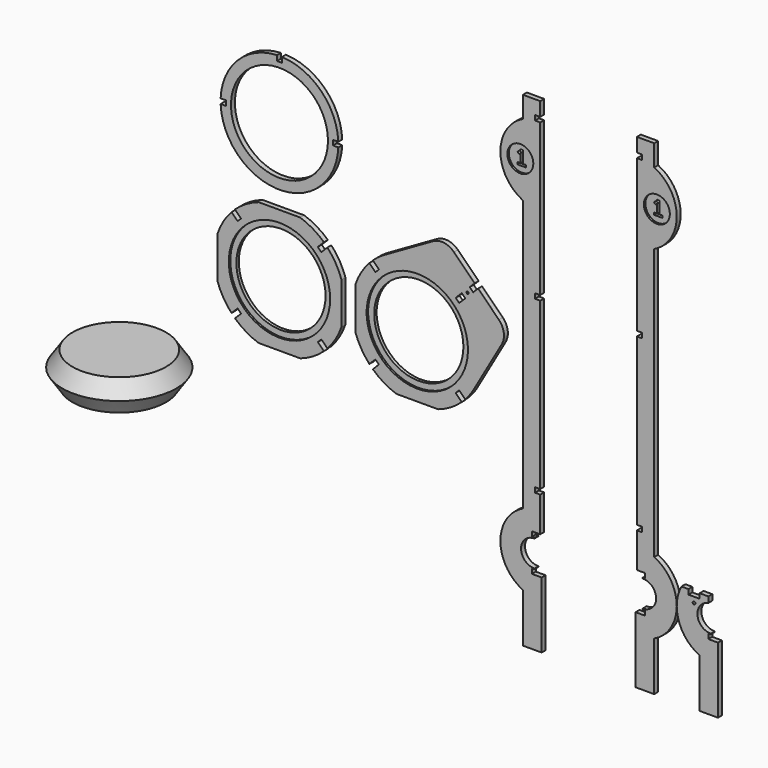
from build123d import *

# Parameters (mm, degrees)
F1_R     = 177.8
F2_DEPTH = 18.034
F1_R_2   = 185.7375
F1_R_3   = 3.81
F1_R_4   = 47.625
F1_W     = 5.08
F1_H     = 242.316
F1_R_5   = 5.08
F1_R_6   = 163.5125
F3_DEPTH = 11.176
F1_W_2   = 171.45
F1_H_2   = 114.3


# Not quite as in the source:
# - a variable given as a bare number and used for a length is read in inches; the dataset says mm whatever the document's units were
# - a feature names something its author has since deleted; it is built from what else it names


with BuildPart() as f2:
    # F1 (on Front) → F2 (new body)
    with BuildSketch(Plane.XZ):
        with BuildLine():
            Line((196.661621641, 517.017), (215.711621641, 517.017))
            ThreePointArc((215.711621641, 517.017), (152.6643540582, 660.6643540582), (9.017, 723.711621641))
            Line((9.017, 723.711621641), (9.017, 704.661621641))
            Line((9.017, 704.661621641), (-9.017, 704.661621641))
            Line((-9.017, 704.661621641), (-9.017, 723.711621641))
            ThreePointArc((-9.017, 723.711621641), (-152.6643540582, 660.6643540582), (-215.711621641, 517.017))
            Line((-215.711621641, 517.017), (-196.661621641, 517.017))
            Line((-196.661621641, 517.017), (-196.661621641, 498.983))
            Line((-196.661621641, 498.983), (-215.711621641, 498.983))
            ThreePointArc((-215.711621641, 498.983), (0, 292.1), (215.711621641, 498.983))
            Line((215.711621641, 498.983), (196.661621641, 498.983))
            Line((196.661621641, 498.983), (196.661621641, 517.017))
        make_face()
        with Locations((0, 508)):
            Circle(F1_R, mode=Mode.SUBTRACT)
    extrude(amount=F2_DEPTH)


with BuildPart() as f2b:
    # F1 (on Front) → F2, piece 2 (new body)
    with BuildSketch(Plane.XZ):
        with BuildLine():
            Line((76.2, 227.2787773996), (-76.2, 227.2787773996))
            ThreePointArc((-76.2, 227.2787773996), (-122.3458738565, 206.1396851811), (-163.0063908604, 175.7583545523))
            Line((-163.0063908604, 175.7583545523), (-140.6757121365, 153.4276758285))
            Line((-140.6757121365, 153.4276758285), (-153.4276758285, 140.6757121365))
            Line((-153.4276758285, 140.6757121365), (-175.7583545523, 163.0063908604))
            ThreePointArc((-175.7583545523, 163.0063908604), (-206.1396851811, 122.3458738565), (-227.2787773996, 76.2))
            Line((-227.2787773996, 76.2), (-227.2787773996, -76.2))
            ThreePointArc((-227.2787773996, -76.2), (-206.1396851811, -122.3458738565), (-175.7583545523, -163.0063908604))
            Line((-175.7583545523, -163.0063908604), (-153.4276758285, -140.6757121365))
            Line((-153.4276758285, -140.6757121365), (-140.6757121365, -153.4276758285))
            Line((-140.6757121365, -153.4276758285), (-163.0063908604, -175.7583545523))
            ThreePointArc((-163.0063908604, -175.7583545523), (-122.3458738565, -206.1396851811), (-76.2, -227.2787773996))
            Line((-76.2, -227.2787773996), (76.2, -227.2787773996))
            ThreePointArc((76.2, -227.2787773996), (122.3458738565, -206.1396851811), (163.0063908604, -175.7583545523))
            Line((163.0063908604, -175.7583545523), (140.6757121365, -153.4276758285))
            Line((140.6757121365, -153.4276758285), (153.4276758285, -140.6757121365))
            Line((153.4276758285, -140.6757121365), (175.7583545523, -163.0063908604))
            ThreePointArc((175.7583545523, -163.0063908604), (206.1396851811, -122.3458738565), (227.2787773996, -76.2))
            Line((227.2787773996, -76.2), (227.2787773996, 76.2))
            ThreePointArc((227.2787773996, 76.2), (206.1396851811, 122.3458738565), (175.7583545523, 163.0063908604))
            Line((175.7583545523, 163.0063908604), (153.4276758285, 140.6757121365))
            Line((153.4276758285, 140.6757121365), (140.6757121365, 153.4276758285))
            Line((140.6757121365, 153.4276758285), (163.0063908604, 175.7583545523))
            ThreePointArc((163.0063908604, 175.7583545523), (122.3458738565, 206.1396851811), (76.2, 227.2787773996))
        make_face()
        Circle(F1_R_2, mode=Mode.SUBTRACT)
    extrude(amount=F2_DEPTH)

    # F1 (on Front) → F3 (join)
    with BuildSketch(Plane.XZ):
        Circle(F1_R_2)
        Circle(F1_R_6, mode=Mode.SUBTRACT)
    extrude(amount=F3_DEPTH)


with BuildPart() as f2c:
    # F1 (on Front) → F2, piece 3 (new body)
    with BuildSketch(Plane.XZ):
        with BuildLine():
            Line((646.0332669357, -153.4276758285), (658.7852306276, -140.6757121365))
            Line((658.7852306276, -140.6757121365), (681.1159093515, -163.0063908604))
            ThreePointArc((681.1159093515, -163.0063908604), (701.321703842, -138.0584475726), (718.0125690949, -110.6342060628))
            ThreePointArc((718.0125690949, -110.6342060628), (725.9972246359, -93.7028214656), (732.6363321988, -76.2))
            Line((732.6363321988, -76.2), (732.6363321988, 76.2))
            ThreePointArc((732.6363321988, 76.2), (711.4972399802, 122.3458738565), (681.1159093515, 163.0063908604))
            Line((681.1159093515, 163.0063908604), (658.7852306276, 140.6757121365))
            Line((658.7852306276, 140.6757121365), (646.0332669357, 153.4276758285))
            Line((646.0332669357, 153.4276758285), (668.3639456595, 175.7583545523))
            ThreePointArc((668.3639456595, 175.7583545523), (627.7034286556, 206.1396851811), (581.5575547992, 227.2787773996))
            Line((581.5575547992, 227.2787773996), (429.1575547992, 227.2787773996))
            ThreePointArc((429.1575547992, 227.2787773996), (411.6547333336, 220.6396698367), (394.7233487364, 212.6550142957))
            ThreePointArc((394.7233487364, 212.6550142957), (367.2991072265, 195.9641490428), (342.3511639388, 175.7583545523))
            Line((342.3511639388, 175.7583545523), (364.6818426626, 153.4276758285))
            Line((364.6818426626, 153.4276758285), (351.9298789707, 140.6757121365))
            Line((351.9298789707, 140.6757121365), (329.5992002469, 163.0063908604))
            ThreePointArc((329.5992002469, 163.0063908604), (299.2178696181, 122.3458738565), (278.0787773996, 76.2))
            Line((278.0787773996, 76.2), (278.0787773996, -76.2))
            ThreePointArc((278.0787773996, -76.2), (299.2178696181, -122.3458738565), (329.5992002469, -163.0063908604))
            Line((329.5992002469, -163.0063908604), (351.9298789707, -140.6757121365))
            Line((351.9298789707, -140.6757121365), (364.6818426626, -153.4276758285))
            Line((364.6818426626, -153.4276758285), (342.3511639388, -175.7583545523))
            ThreePointArc((342.3511639388, -175.7583545523), (383.0116809427, -206.1396851811), (429.1575547992, -227.2787773996))
            Line((429.1575547992, -227.2787773996), (581.5575547992, -227.2787773996))
            ThreePointArc((581.5575547992, -227.2787773996), (627.7034286556, -206.1396851811), (668.3639456595, -175.7583545523))
            Line((668.3639456595, -175.7583545523), (646.0332669357, -153.4276758285))
        make_face()
        with Locations((505.3575547992, 0)):
            Circle(F1_R_2, mode=Mode.SUBTRACT)
        with BuildLine():
            ThreePointArc((732.6363321988, -76.2), (725.9972246359, -93.7028214656), (718.0125690949, -110.6342060628))
            Line((718.0125690949, -110.6342060628), (814.5833852283, 57.7646913023))
            ThreePointArc((814.5833852283, 57.7646913023), (822.4429089781, 97.7343199195), (804.399605341, 134.2553072998))
            Line((804.399605341, 134.2553072998), (728.3822155659, 210.2726970748))
            Line((728.3822155659, 210.2726970748), (710.3017417449, 192.1922232538))
            Line((710.3017417449, 192.1922232538), (697.549778053, 204.9441869458))
            Line((697.549778053, 204.9441869458), (715.630251874, 223.0246607668))
            Line((715.630251874, 223.0246607668), (639.612862099, 299.0420505418))
            ThreePointArc((639.612862099, 299.0420505418), (603.0918747187, 317.085354179), (563.1222461014, 309.2258304291))
            Line((563.1222461014, 309.2258304291), (394.7233487364, 212.6550142957))
            ThreePointArc((394.7233487364, 212.6550142957), (411.6547333336, 220.6396698367), (429.1575547992, 227.2787773996))
            Line((429.1575547992, 227.2787773996), (581.5575547992, 227.2787773996))
            ThreePointArc((581.5575547992, 227.2787773996), (627.7034286556, 206.1396851811), (668.3639456595, 175.7583545523))
            ThreePointArc((668.3639456595, 175.7583545523), (674.8598890843, 169.5023342852), (681.1159093515, 163.0063908604))
            ThreePointArc((681.1159093515, 163.0063908604), (711.4972399802, 122.3458738565), (732.6363321988, 76.2))
            Line((732.6363321988, 76.2), (732.6363321988, -76.2))
        make_face()
        with Locations((689.3928244917, 184.0352696925)):
            Circle(F1_R_3, mode=Mode.SUBTRACT)
    extrude(amount=F2_DEPTH)

    # F1 (on Front) → F3, piece 2 (join)
    with BuildSketch(Plane.XZ):
        with Locations((505.3575547992, 0)):
            Circle(F1_R_2)
        with Locations((505.3575547992, 0)):
            Circle(F1_R_6, mode=Mode.SUBTRACT)
    extrude(amount=F3_DEPTH)


with BuildPart() as f2d:
    # F1 (on Front) → F2, piece 4 (new body)
    with BuildSketch(Plane.XZ):
        with BuildLine():
            Line((1373.9863321988, 889), (1310.4863321988, 889))
            Line((1310.4863321988, 889), (1310.4863321988, 838.2))
            Line((1310.4863321988, 838.2), (1329.5363321988, 838.2))
            Line((1329.5363321988, 838.2), (1329.5363321988, 820.166))
            Line((1329.5363321988, 820.166), (1310.4863321988, 820.166))
            Line((1310.4863321988, 820.166), (1310.4863321988, 263.017))
            Line((1310.4863321988, 263.017), (1329.5363321988, 263.017))
            Line((1329.5363321988, 263.017), (1329.5363321988, 244.983))
            Line((1329.5363321988, 244.983), (1310.4863321988, 244.983))
            Line((1310.4863321988, 244.983), (1310.4863321988, -362.966))
            Line((1310.4863321988, -362.966), (1329.5363321988, -362.966))
            Line((1329.5363321988, -362.966), (1329.5363321988, -381))
            Line((1329.5363321988, -381), (1310.4863321988, -381))
            Line((1310.4863321988, -381), (1310.4863321988, -487.934))
            Line((1310.4863321988, -487.934), (1310.4863321988, -509.016))
            Line((1310.4863321988, -509.016), (1340.8367921988, -509.016))
            Line((1340.8367921988, -509.016), (1340.8367921988, -527.05))
            Line((1340.8367921988, -527.05), (1331.7029521988, -527.05))
            Line((1331.7029521988, -527.05), (1331.7029521988, -529.6289769048))
            ThreePointArc((1331.7029521988, -529.6289769048), (1380.8443321988, -577.85), (1331.7029521988, -626.0710230952))
            Line((1331.7029521988, -626.0710230952), (1331.7029521988, -628.65))
            Line((1331.7029521988, -628.65), (1340.8367921988, -628.65))
            Line((1340.8367921988, -628.65), (1340.8367921988, -646.684))
            Line((1340.8367921988, -646.684), (1310.4863321988, -646.684))
            Line((1310.4863321988, -646.684), (1310.4863321988, -889))
            Line((1310.4863321988, -889), (1373.9863321988, -889))
            Line((1373.9863321988, -889), (1373.9863321988, -709.3732013753))
            ThreePointArc((1373.9863321988, -709.3732013753), (1434.18915654, -655.491572305), (1456.5363321988, -577.85))
            ThreePointArc((1456.5363321988, -577.85), (1434.18915654, -500.208427695), (1373.9863321988, -446.3267986247))
            Line((1373.9863321988, -446.3267986247), (1373.9863321988, 547.9267986247))
            ThreePointArc((1373.9863321988, 547.9267986247), (1456.5363321988, 679.45), (1373.9863321988, 810.9732013753))
            Line((1373.9863321988, 810.9732013753), (1373.9863321988, 889))
        make_face()
        with Locations((1383.5113321988, 679.45)):
            Circle(F1_R_4, mode=Mode.SUBTRACT)
        with Locations((1307.9463321988, -767.842)):
            Rectangle(F1_W, F1_H)
    extrude(amount=F2_DEPTH)

    # F1 (on Front) → F3, piece 3 (join)
    with BuildSketch(Plane.XZ):
        with Locations((1383.5113321988, 679.45)):
            Circle(F1_R_4)
        Polygon((1379.3838321988, 705.8025), (1387.6388321988, 705.8025), (1387.6388321988, 661.3525), (1399.3863321988, 661.3525), (1399.3863321988, 653.0975), (1367.6363321988, 653.0975), (1367.6363321988, 661.3525), (1379.3838321988, 661.3525), (1379.3838321988, 693.9693540915), (1373.5508018566, 687.9786742806), (1367.6363321988, 693.7375), align=None, mode=Mode.SUBTRACT)
    extrude(amount=F3_DEPTH)


with BuildPart() as f2e:
    # F1 (on Front) → F2, piece 5 (new body)
    with BuildSketch(Plane.XZ):
        with BuildLine():
            Line((936.9945721988, 838.2), (956.0445721988, 838.2))
            Line((956.0445721988, 838.2), (956.0445721988, 889))
            Line((956.0445721988, 889), (892.5445721988, 889))
            Line((892.5445721988, 889), (892.5445721988, 810.9732013753))
            ThreePointArc((892.5445721988, 810.9732013753), (809.9945721988, 679.45), (892.5445721988, 547.9267986247))
            Line((892.5445721988, 547.9267986247), (892.5445721988, -446.3267986247))
            ThreePointArc((892.5445721988, -446.3267986247), (809.9945721988, -577.85), (892.5445721988, -709.3732013753))
            Line((892.5445721988, -709.3732013753), (892.5445721988, -889))
            Line((892.5445721988, -889), (956.0445721988, -889))
            Line((956.0445721988, -889), (956.0445721988, -646.684))
            Line((956.0445721988, -646.684), (925.6941121988, -646.684))
            Line((925.6941121988, -646.684), (925.6941121988, -628.65))
            Line((925.6941121988, -628.65), (934.8279521988, -628.65))
            Line((934.8279521988, -628.65), (934.8279521988, -626.0710230952))
            ThreePointArc((934.8279521988, -626.0710230952), (885.6865721988, -577.85), (934.8279521988, -529.6289769048))
            Line((934.8279521988, -529.6289769048), (934.8279521988, -527.05))
            Line((934.8279521988, -527.05), (925.6941121988, -527.05))
            Line((925.6941121988, -527.05), (925.6941121988, -509.016))
            Line((925.6941121988, -509.016), (956.0445721988, -509.016))
            Line((956.0445721988, -509.016), (956.0445721988, -487.934))
            Line((956.0445721988, -487.934), (956.0445721988, -381))
            Line((956.0445721988, -381), (936.9945721988, -381))
            Line((936.9945721988, -381), (936.9945721988, -362.966))
            Line((936.9945721988, -362.966), (956.0445721988, -362.966))
            Line((956.0445721988, -362.966), (956.0445721988, 244.983))
            Line((956.0445721988, 244.983), (936.9945721988, 244.983))
            Line((936.9945721988, 244.983), (936.9945721988, 263.017))
            Line((936.9945721988, 263.017), (956.0445721988, 263.017))
            Line((956.0445721988, 263.017), (956.0445721988, 820.166))
            Line((956.0445721988, 820.166), (936.9945721988, 820.166))
            Line((936.9945721988, 820.166), (936.9945721988, 838.2))
        make_face()
        with Locations((883.0195721988, 679.45)):
            Circle(F1_R_4, mode=Mode.SUBTRACT)
        with Locations((958.5845721988, -767.842)):
            Rectangle(F1_W, F1_H)
    extrude(amount=F2_DEPTH)

    # F1 (on Front) → F3, piece 4 (join)
    with BuildSketch(Plane.XZ):
        with Locations((883.0195721988, 679.45)):
            Circle(F1_R_4)
        Polygon((878.8920721988, 705.8025), (887.1470721988, 705.8025), (887.1470721988, 661.3525), (898.8945721988, 661.3525), (898.8945721988, 653.0975), (867.1445721988, 653.0975), (867.1445721988, 661.3525), (878.8920721988, 661.3525), (878.8920721988, 693.9693540915), (873.0590418566, 687.9786742806), (867.1445721988, 693.7375), align=None, mode=Mode.SUBTRACT)
    extrude(amount=F3_DEPTH)


with BuildPart() as f2f:
    # F1 (on Front) → F2, piece 6 (new body)
    with BuildSketch(Plane.XZ):
        with BuildLine():
            ThreePointArc((1473.7745200696, -509.016), (1460.9114091152, -542.3701653151), (1456.5363321988, -577.85))
            ThreePointArc((1456.5363321988, -577.85), (1478.8835078575, -655.491572305), (1539.0863321988, -709.3732013753))
            Line((1539.0863321988, -709.3732013753), (1539.0863321988, -889))
            Line((1539.0863321988, -889), (1602.5863321988, -889))
            Line((1602.5863321988, -889), (1607.6663321988, -889))
            Line((1607.6663321988, -889), (1607.6663321988, -646.684))
            Line((1607.6663321988, -646.684), (1602.5863321988, -646.684))
            Line((1602.5863321988, -646.684), (1572.2358721988, -646.684))
            Line((1572.2358721988, -646.684), (1572.2358721988, -628.65))
            Line((1572.2358721988, -628.65), (1581.3697121988, -628.65))
            Line((1581.3697121988, -628.65), (1581.3697121988, -626.0710230952))
            ThreePointArc((1581.3697121988, -626.0710230952), (1532.4463087452, -582.4302126234), (1572.2358721988, -530.3263703054))
            Line((1572.2358721988, -530.3263703054), (1572.2358721988, -527.05))
            Line((1572.2358721988, -527.05), (1572.2358721988, -509.016))
            Line((1572.2358721988, -509.016), (1540.4858721988, -509.016))
            Line((1540.4858721988, -509.016), (1540.4858721988, -527.05))
            Line((1540.4858721988, -527.05), (1499.2108721988, -527.05))
            Line((1499.2108721988, -527.05), (1499.2108721988, -509.016))
            Line((1499.2108721988, -509.016), (1473.7745200696, -509.016))
        make_face()
        with Locations((1519.8483721988, -547.37)):
            Circle(F1_R_5, mode=Mode.SUBTRACT)
    extrude(amount=F2_DEPTH)


with BuildPart() as f4:
    # F1 (on Front) → F4 (revolve)
    with BuildSketch(Plane.XZ):
        with Locations((-515.9585163116, -483.864790535)):
            Rectangle(F1_W_2, F1_H_2)
        Polygon((-392.1335163116, -483.864790535), (-430.2335163116, -426.714790535), (-430.2335163116, -541.014790535), align=None)
    revolve(axis=Axis((-601.6835163116, 0, -483.864790535), (0, 0, -1)))


solid = Compound([f2.part, f2b.part, f2c.part, f2d.part, f2e.part, f2f.part, f4.part])
